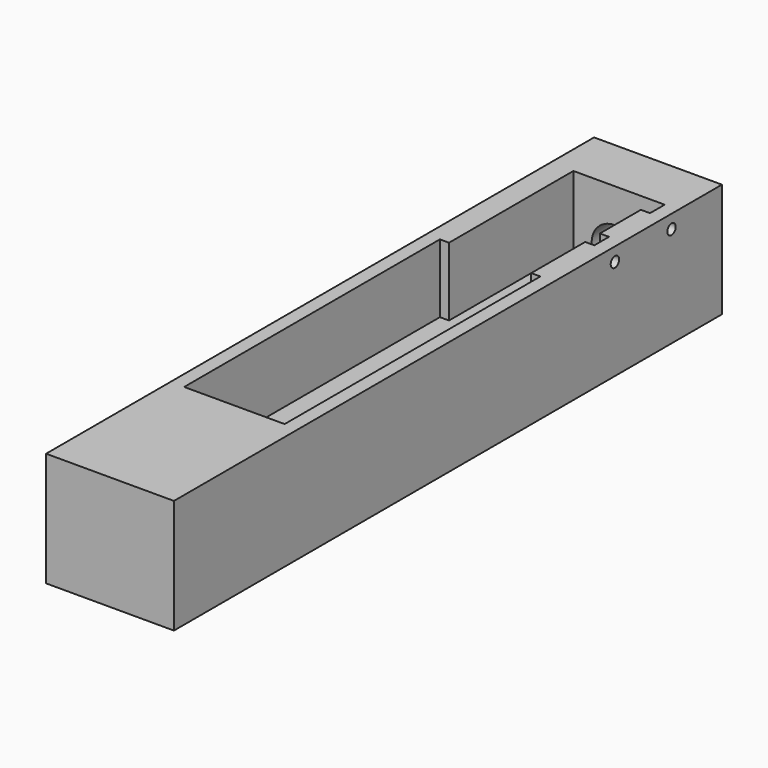
from build123d import *

# Parameters (mm, degrees)
F0_W      = 28
F0_H      = 25
F1_DEPTH  = 150
F2_R      = 9.525
F3_DEPTH  = 17
F4_R      = 1.5
F5_DEPTH  = 5
F6_R      = 1.5
F7_DEPTH  = 25.001
F8_W      = 22
F8_H      = 70
F9_DEPTH  = 15
F10_R     = 1.15
F11_DEPTH = 5
F12_W     = 2
F12_H     = 4.0241825168
F13_DEPTH = 5
F14_W     = 18
F14_H     = 19.2723592291
F15_DEPTH = 15
F16_W     = 18
F16_H     = 14.7685540254
F17_DEPTH = 15
F18_R     = 5
F19_DEPTH = 12


# Not quite as in the source:
# - the program builds the solid bodies; features that only make, move or delete a surface that nothing else refers to are left out


with BuildPart() as f1:
    # F0 (on Front) → F1 (new body)
    with BuildSketch(Plane.XZ):
        Rectangle(F0_W, F0_H)
    extrude(amount=-F1_DEPTH)

    # F2 (on face) → F3 (cut)
    with BuildSketch(Plane(origin=(0, 0, -12.5), x_dir=(1, 0, 0), z_dir=(0, 0, -1))):
        with Locations((0, -14.525)):
            Circle(F2_R)
    extrude(amount=-F3_DEPTH, mode=Mode.SUBTRACT)

    # F4 (on face) → F5 (cut)
    with BuildSketch(Plane(origin=(0, 0, -12.5), x_dir=(1, 0, 0), z_dir=(0, 0, -1))):
        with BuildLine():
            ThreePointArc((1.6602502077, -54.4256372334), (2.8756374132, -53.2102498962), (3.3205, -51.55))
            ThreePointArc((3.3205, -51.55), (2.8756373339, -49.8897499664), (1.6602499328, -48.6743626079))
            ThreePointArc((1.6602499328, -48.6743626079), (-1.397e-07, -48.2295), (-1.6602501748, -48.6743627476))
            ThreePointArc((-1.6602501748, -48.6743627476), (-2.8756374037, -49.8897500874), (-3.3205, -51.55))
            ThreePointArc((-3.3205, -51.55), (-2.8756373712, -53.210249969), (-1.660250062, -54.4256373175))
            ThreePointArc((-1.660250062, -54.4256373175), (8.41e-08, -54.8705), (1.6602502077, -54.4256372334))
        make_face()
        with Locations((0, -51.55)):
            Circle(F4_R, mode=Mode.SUBTRACT)
        with BuildLine():
            Line((3.3205, -53.4670915688), (3.3205, -51.55))
            ThreePointArc((3.3205, -51.55), (2.8756374132, -53.2102498962), (1.6602502077, -54.4256372334))
            Line((1.6602502077, -54.4256372334), (3.3205, -53.4670915688))
        make_face()
        with BuildLine():
            ThreePointArc((1.6602499328, -48.6743626079), (2.8756373339, -49.8897499664), (3.3205, -51.55))
            Line((3.3205, -51.55), (3.3205, -49.6329084312))
            Line((3.3205, -49.6329084312), (1.6602499328, -48.6743626079))
        make_face()
        with BuildLine():
            ThreePointArc((-1.6602501748, -48.6743627476), (-1.397e-07, -48.2295), (1.6602499328, -48.6743626079))
            Line((1.6602499328, -48.6743626079), (0, -47.7158168623))
            Line((0, -47.7158168623), (-1.6602501748, -48.6743627476))
        make_face()
        with BuildLine():
            Line((0, -55.3841831377), (1.6602502077, -54.4256372334))
            ThreePointArc((1.6602502077, -54.4256372334), (8.41e-08, -54.8705), (-1.660250062, -54.4256373175))
            Line((-1.660250062, -54.4256373175), (0, -55.3841831377))
        make_face()
        with BuildLine():
            ThreePointArc((-3.3205, -51.55), (-2.8756374037, -49.8897500874), (-1.6602501748, -48.6743627476))
            Line((-1.6602501748, -48.6743627476), (-3.3205, -49.6329084312))
            Line((-3.3205, -49.6329084312), (-3.3205, -51.55))
        make_face()
        with BuildLine():
            Line((-3.3205, -53.4670915688), (-1.660250062, -54.4256373175))
            ThreePointArc((-1.660250062, -54.4256373175), (-2.8756373712, -53.210249969), (-3.3205, -51.55))
            Line((-3.3205, -51.55), (-3.3205, -53.4670915688))
        make_face()
        with BuildLine():
            ThreePointArc((1.6602500198, -89.4256373418), (2.875637359, -88.2102499901), (3.3205, -86.55))
            ThreePointArc((3.3205, -86.55), (2.8756374351, -84.8897501418), (1.6602502837, -83.6743628105))
            ThreePointArc((1.6602502837, -83.6743628105), (-2.2e-09, -83.2295), (-1.6602502875, -83.6743628127))
            ThreePointArc((-1.6602502875, -83.6743628127), (-2.8756374363, -84.8897501438), (-3.3205, -86.55))
            ThreePointArc((-3.3205, -86.55), (-2.875637359, -88.2102499901), (-1.6602500198, -89.4256373418))
            ThreePointArc((-1.6602500198, -89.4256373418), (0, -89.8705), (1.6602500198, -89.4256373418))
        make_face()
        with Locations((0, -86.55)):
            Circle(F4_R, mode=Mode.SUBTRACT)
        with BuildLine():
            Line((3.3205, -88.4670915688), (3.3205, -86.55))
            ThreePointArc((3.3205, -86.55), (2.875637359, -88.2102499901), (1.6602500198, -89.4256373418))
            Line((1.6602500198, -89.4256373418), (3.3205, -88.4670915688))
        make_face()
        with BuildLine():
            ThreePointArc((1.6602502837, -83.6743628105), (2.8756374351, -84.8897501418), (3.3205, -86.55))
            Line((3.3205, -86.55), (3.3205, -84.6329084312))
            Line((3.3205, -84.6329084312), (1.6602502837, -83.6743628105))
        make_face()
        with BuildLine():
            ThreePointArc((-1.6602502875, -83.6743628127), (-2.2e-09, -83.2295), (1.6602502837, -83.6743628105))
            Line((1.6602502837, -83.6743628105), (0, -82.7158168623))
            Line((0, -82.7158168623), (-1.6602502875, -83.6743628127))
        make_face()
        with BuildLine():
            Line((0, -90.3841831377), (1.6602500198, -89.4256373418))
            ThreePointArc((1.6602500198, -89.4256373418), (0, -89.8705), (-1.6602500198, -89.4256373418))
            Line((-1.6602500198, -89.4256373418), (0, -90.3841831377))
        make_face()
        with BuildLine():
            ThreePointArc((-3.3205, -86.55), (-2.8756374363, -84.8897501438), (-1.6602502875, -83.6743628127))
            Line((-1.6602502875, -83.6743628127), (-3.3205, -84.6329084312))
            Line((-3.3205, -84.6329084312), (-3.3205, -86.55))
        make_face()
        with BuildLine():
            Line((-3.3205, -88.4670915688), (-1.6602500198, -89.4256373418))
            ThreePointArc((-1.6602500198, -89.4256373418), (-2.875637359, -88.2102499901), (-3.3205, -86.55))
            Line((-3.3205, -86.55), (-3.3205, -88.4670915688))
        make_face()
    extrude(amount=-F5_DEPTH, mode=Mode.SUBTRACT)

    # F6 (on face) → F7 (cut, through all)
    with BuildSketch(Plane(origin=(0, 0, -12.5), x_dir=(1, 0, 0), z_dir=(0, 0, -1))):
        with Locations((0, -51.55)):
            Circle(F6_R)
        with Locations((0, -86.55)):
            Circle(F6_R)
    extrude(amount=-F7_DEPTH, mode=Mode.SUBTRACT)

    # F8 (on face) → F9 (cut)
    with BuildSketch(Plane.XY.offset(12.5)):
        with Locations((0, 69.05)):
            Rectangle(F8_W, F8_H)
    extrude(amount=-F9_DEPTH, mode=Mode.SUBTRACT)

    # F10 (on face) → F11 (cut)
    with BuildSketch(Plane.YZ.offset(14)):
        with Locations((136.2115726471, 9.5113839224)):
            Circle(F10_R)
        with Locations((120.7115726471, 9.5113839224)):
            Circle(F10_R)
    extrude(amount=-F11_DEPTH, mode=Mode.SUBTRACT)

    # F12 (on face) → F13 (cut)
    with BuildSketch(Plane.XY.offset(12.5)):
        with Locations((10, 120.8306452838)):
            Rectangle(F12_W, F12_H)
        with Locations((10, 136.0788219961)):
            Rectangle(F12_W, F12_H)
    extrude(amount=-F13_DEPTH, mode=Mode.SUBTRACT)

    # F14 (on face) → F15 (cut)
    with BuildSketch(Plane.XY.offset(12.5)):
        with Locations((0, 128.45473364)):
            Rectangle(F14_W, F14_H)
    extrude(amount=-F15_DEPTH, mode=Mode.SUBTRACT)

    # F16 (on face) → F17 (cut)
    with BuildSketch(Plane.XY.offset(12.5)):
        with Locations((0, 111.4342770127)):
            Rectangle(F16_W, F16_H)
    extrude(amount=-F17_DEPTH, mode=Mode.SUBTRACT)

    # F18 (on face) → F19 (cut)
    with BuildSketch(Plane(origin=(0, 150, 0), x_dir=(-1, 0, 0), z_dir=(0, 1, 0))):
        Circle(F18_R)
    extrude(amount=-F19_DEPTH, mode=Mode.SUBTRACT)


solid = f1.part
